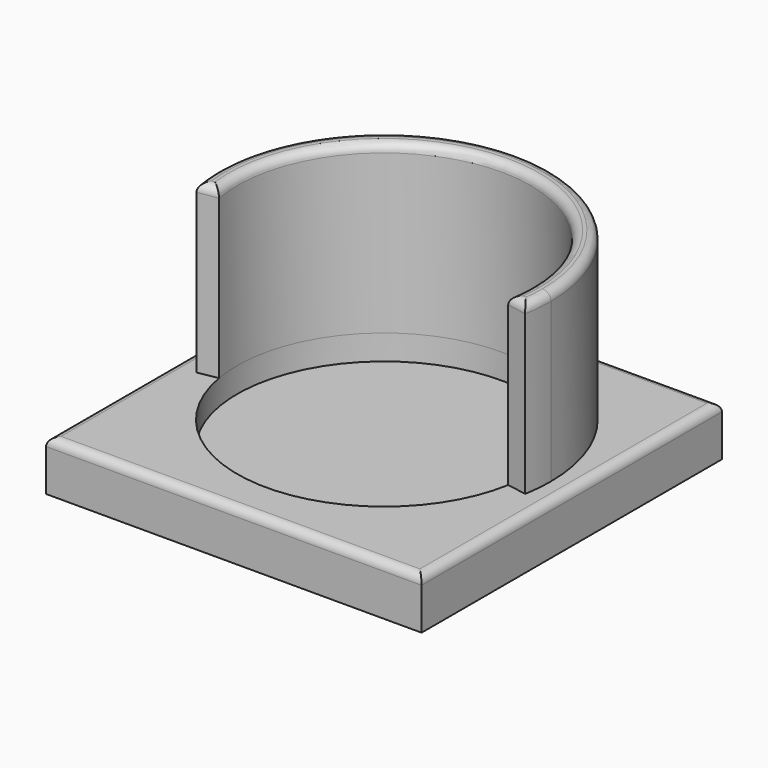
from build123d import *
from build123d import SkipClean  # not in build123d's __all__

# Parameters (mm, degrees)
F0_W     = 45
F0_H     = 45
F1_DEPTH = 6
F2_R     = 17.6
F3_DEPTH = 3
F5_DEPTH = 20
F6_R     = 1


with BuildPart() as f1:
    # F0 (on Top) → F1 (new body)
    with BuildSketch(Plane.XY):
        Rectangle(F0_W, F0_H)
    extrude(amount=F1_DEPTH)

    # F2 (on face) → F3 (cut)
    with BuildSketch(Plane.XY.offset(6)):
        Circle(F2_R)
    extrude(amount=-F3_DEPTH, mode=Mode.SUBTRACT)

    # F4 (on face) → F5 (join)
    with BuildSketch(Plane.XY.offset(6)):
        with BuildLine():
            ThreePointArc((19.696155, -3.472964), (19.923894, -1.743115), (20, 0))
            ThreePointArc((20, 0), (-1.743115, 19.923894), (-19.696155, -3.472964))
            Line((-19.696155, -3.472964), (-17.332616, -3.056208))
            ThreePointArc((-17.332616, -3.056208), (-1.533941, 17.533027), (17.6, 0))
            ThreePointArc((17.6, 0), (17.533027, -1.533941), (17.332616, -3.056208))
            Line((17.332616, -3.056208), (19.696155, -3.472964))
        make_face()
    with SkipClean():  # cleaning this boolean's faces spoils the solid; the shape is the same uncleaned
        extrude(amount=F5_DEPTH)

    # F6
    f6_edges = [f1.edges().sort_by_distance(p)[0] for p in [
        (0, -22.5, 6),
        (22.5, 0, 6),
        (0, 22.5, 6),
        (-22.5, 0, 6),
        (-1.533941, 17.533027, 26),
        (0, 20, 26),
        (-18.514386, -3.264586, 26),
        (18.514386, -3.264586, 26),
    ]]
    fillet(f6_edges, radius=F6_R)


solid = f1.part
